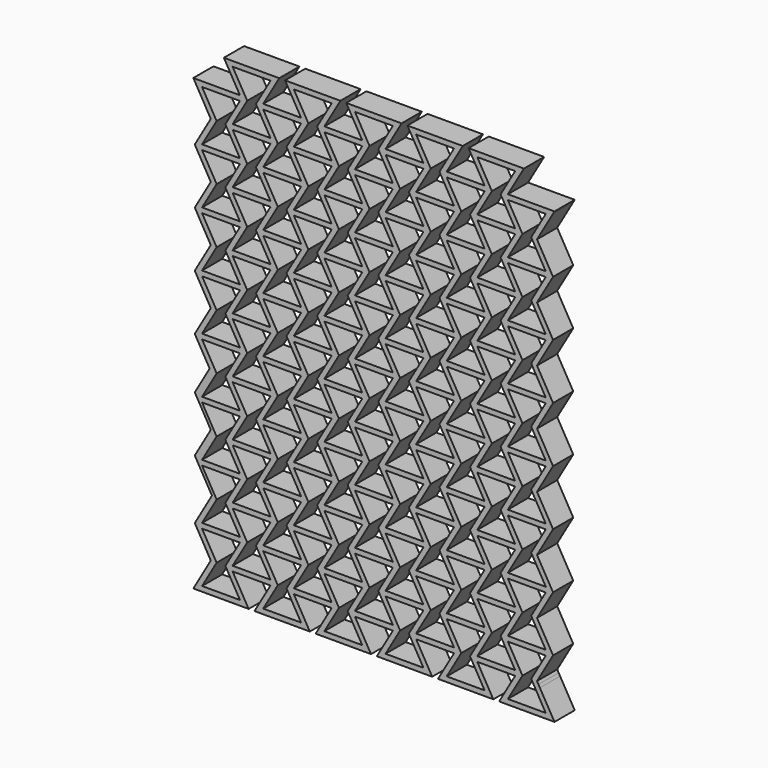
from build123d import *

# Parameters (mm, degrees)
F0_W     = 212.4550379813
F0_H     = 214.7212279961
F1_DEPTH = 10
F2_W     = 316.5591433644
F2_H     = 238.5154794902
F3_DEPTH = 50


# Not quite as in the source:
# - ends of sketch curves that miss each other by under 0.0002 mm in the source are joined


with BuildPart() as f1:
    # F0 (on Front) → F1 (new body)
    with BuildSketch(Plane.XZ):
        with Locations((69.8008518666, 93.7357270159)):
            Rectangle(F0_W, F0_H)
        Polygon((15, 0), (0, 0), (5.7735026919, 10), (0, 20), (15, 20), (9.2264973081, 10), align=None, mode=Mode.SUBTRACT)
        Polygon((15, 22), (0, 22), (5.7735026919, 32), (0, 42), (15, 42), (9.2264973081, 32), align=None, mode=Mode.SUBTRACT)
        Polygon((39.2264973081, 0), (24.2264973081, 0), (30, 10), (24.2264973081, 20), (39.2264973081, 20), (33.4529946162, 10), align=None, mode=Mode.SUBTRACT)
        Polygon((63.4529946162, 0), (48.4529946162, 0), (54.2264973081, 10), (48.4529946162, 20), (63.4529946162, 20), (57.6794919243, 10), align=None, mode=Mode.SUBTRACT)
        Polygon((27.1132486541, 11), (12.1132486541, 11), (17.8867513459, 21), (12.1132486541, 31), (27.1132486541, 31), (21.3397459622, 21), align=None, mode=Mode.SUBTRACT)
        Polygon((39.2264973081, 22), (24.2264973081, 22), (30, 32), (24.2264973081, 42), (39.2264973081, 42), (33.4529946162, 32), align=None, mode=Mode.SUBTRACT)
        Polygon((51.3397459622, 11), (36.3397459622, 11), (42.1132486541, 21), (36.3397459622, 31), (51.3397459622, 31), (45.5662432703, 21), align=None, mode=Mode.SUBTRACT)
        Polygon((75.5662432703, 11), (60.5662432703, 11), (66.3397459622, 21), (60.5662432703, 31), (75.5662432703, 31), (69.7927405784, 21), align=None, mode=Mode.SUBTRACT)
        Polygon((63.4529946162, 22), (48.4529946162, 22), (54.2264973081, 32), (48.4529946162, 42), (63.4529946162, 42), (57.6794919243, 32), align=None, mode=Mode.SUBTRACT)
        Polygon((15, 44), (0, 44), (5.7735026919, 54), (0, 64), (15, 64), (9.2264973081, 54), align=None, mode=Mode.SUBTRACT)
        Polygon((15, 66), (0, 66), (5.7735026919, 76), (0, 86), (15, 86), (9.2264973081, 76), align=None, mode=Mode.SUBTRACT)
        Polygon((27.1132486541, 33), (12.1132486541, 33), (17.8867513459, 43), (12.1132486541, 53), (27.1132486541, 53), (21.3397459622, 43), align=None, mode=Mode.SUBTRACT)
        Polygon((27.1132486541, 55), (12.1132486541, 55), (17.8867513459, 65), (12.1132486541, 75), (27.1132486541, 75), (21.3397459622, 65), align=None, mode=Mode.SUBTRACT)
        Polygon((39.2264973081, 44), (24.2264973081, 44), (30, 54), (24.2264973081, 64), (39.2264973081, 64), (33.4529946162, 54), align=None, mode=Mode.SUBTRACT)
        Polygon((51.3397459622, 33), (36.3397459622, 33), (42.1132486541, 43), (36.3397459622, 53), (51.3397459622, 53), (45.5662432703, 43), align=None, mode=Mode.SUBTRACT)
        Polygon((75.5662432703, 33), (60.5662432703, 33), (66.3397459622, 43), (60.5662432703, 53), (75.5662432703, 53), (69.7927405784, 43), align=None, mode=Mode.SUBTRACT)
        Polygon((63.4529946162, 44), (48.4529946162, 44), (54.2264973081, 54), (48.4529946162, 64), (63.4529946162, 64), (57.6794919243, 54), align=None, mode=Mode.SUBTRACT)
        Polygon((51.3397459622, 55), (36.3397459622, 55), (42.1132486541, 65), (36.3397459622, 75), (51.3397459622, 75), (45.5662432703, 65), align=None, mode=Mode.SUBTRACT)
        Polygon((75.5662432703, 55), (60.5662432703, 55), (66.3397459622, 65), (60.5662432703, 75), (75.5662432703, 75), (69.7927405784, 65), align=None, mode=Mode.SUBTRACT)
        Polygon((39.2264973081, 66), (24.2264973081, 66), (30, 76), (24.2264973081, 86), (39.2264973081, 86), (33.4529946162, 76), align=None, mode=Mode.SUBTRACT)
        Polygon((27.1132486541, 77), (12.1132486541, 77), (17.8867513459, 87), (12.1132486541, 97), (27.1132486541, 97), (21.3397459622, 87), align=None, mode=Mode.SUBTRACT)
        Polygon((63.4529946162, 66), (48.4529946162, 66), (54.2264973081, 76), (48.4529946162, 86), (63.4529946162, 86), (57.6794919243, 76), align=None, mode=Mode.SUBTRACT)
        Polygon((51.3397459622, 77), (36.3397459622, 77), (42.1132486541, 87), (36.3397459622, 97), (51.3397459622, 97), (45.5662432703, 87), align=None, mode=Mode.SUBTRACT)
        Polygon((75.5662432703, 77), (60.5662432703, 77), (66.3397459622, 87), (60.5662432703, 97), (75.5662432703, 97), (69.7927405784, 87), align=None, mode=Mode.SUBTRACT)
        Polygon((87.6794919243, 0), (72.6794919243, 0), (78.4529946162, 10), (72.6794919243, 20), (87.6794919243, 20), (81.9059892324, 10), align=None, mode=Mode.SUBTRACT)
        Polygon((111.9059892324, 0), (96.9059892324, 0), (102.6794919243, 10), (96.9059892324, 20), (111.9059892324, 20), (106.1324865405, 10), align=None, mode=Mode.SUBTRACT)
        Polygon((99.7927405784, 11), (84.7927405784, 11), (90.5662432703, 21), (84.7927405784, 31), (99.7927405784, 31), (94.0192378865, 21), align=None, mode=Mode.SUBTRACT)
        Polygon((87.6794919243, 22), (72.6794919243, 22), (78.4529946162, 32), (72.6794919243, 42), (87.6794919243, 42), (81.9059892324, 32), align=None, mode=Mode.SUBTRACT)
        Polygon((124.0192378865, 11), (109.0192378865, 11), (114.7927405784, 21), (109.0192378865, 31), (124.0192378865, 31), (118.2457351946, 21), align=None, mode=Mode.SUBTRACT)
        Polygon((111.9059892324, 22), (96.9059892324, 22), (102.6794919243, 32), (96.9059892324, 42), (111.9059892324, 42), (106.1324865405, 32), align=None, mode=Mode.SUBTRACT)
        Polygon((136.1324865405, 0), (121.1324865405, 0), (126.9059892324, 10), (121.1324865405, 20), (136.1324865405, 20), (130.3589838486, 10), align=None, mode=Mode.SUBTRACT)
        Polygon((148.2457351946, 11), (133.2457351946, 11), (139.0192378865, 21), (133.2457351946, 31), (148.2457351946, 31), (142.4722325027, 21), align=None, mode=Mode.SUBTRACT)
        Polygon((136.1324865405, 22), (121.1324865405, 22), (126.9059892324, 32), (121.1324865405, 42), (136.1324865405, 42), (130.3589838486, 32), align=None, mode=Mode.SUBTRACT)
        Polygon((99.7927405784, 33), (84.7927405784, 33), (90.5662432703, 43), (84.7927405784, 53), (99.7927405784, 53), (94.0192378865, 43), align=None, mode=Mode.SUBTRACT)
        Polygon((87.6794919243, 44), (72.6794919243, 44), (78.4529946162, 54), (72.6794919243, 64), (87.6794919243, 64), (81.9059892324, 54), align=None, mode=Mode.SUBTRACT)
        Polygon((99.7927405784, 55), (84.7927405784, 55), (90.5662432703, 65), (84.7927405784, 75), (99.7927405784, 75), (94.0192378865, 65), align=None, mode=Mode.SUBTRACT)
        Polygon((124.0192378865, 33), (109.0192378865, 33), (114.7927405784, 43), (109.0192378865, 53), (124.0192378865, 53), (118.2457351946, 43), align=None, mode=Mode.SUBTRACT)
        Polygon((111.9059892324, 44), (96.9059892324, 44), (102.6794919243, 54), (96.9059892324, 64), (111.9059892324, 64), (106.1324865405, 54), align=None, mode=Mode.SUBTRACT)
        Polygon((124.0192378865, 55), (109.0192378865, 55), (114.7927405784, 65), (109.0192378865, 75), (124.0192378865, 75), (118.2457351946, 65), align=None, mode=Mode.SUBTRACT)
        Polygon((87.6794919243, 66), (72.6794919243, 66), (78.4529946162, 76), (72.6794919243, 86), (87.6794919243, 86), (81.9059892324, 76), align=None, mode=Mode.SUBTRACT)
        Polygon((99.7927405784, 77), (84.7927405784, 77), (90.5662432703, 87), (84.7927405784, 97), (99.7927405784, 97), (94.0192378865, 87), align=None, mode=Mode.SUBTRACT)
        Polygon((111.9059892324, 66), (96.9059892324, 66), (102.6794919243, 76), (96.9059892324, 86), (111.9059892324, 86), (106.1324865405, 76), align=None, mode=Mode.SUBTRACT)
        Polygon((124.0192378865, 77), (109.0192378865, 77), (114.7927405784, 87), (109.0192378865, 97), (124.0192378865, 97), (118.2457351946, 87), align=None, mode=Mode.SUBTRACT)
        Polygon((148.2457351946, 33), (133.2457351946, 33), (139.0192378865, 43), (133.2457351946, 53), (148.2457351946, 53), (142.4722325027, 43), align=None, mode=Mode.SUBTRACT)
        Polygon((136.1324865405, 44), (121.1324865405, 44), (126.9059892324, 54), (121.1324865405, 64), (136.1324865405, 64), (130.3589838486, 54), align=None, mode=Mode.SUBTRACT)
        Polygon((148.2457351946, 55), (133.2457351946, 55), (139.0192378865, 65), (133.2457351946, 75), (148.2457351946, 75), (142.4722325027, 65), align=None, mode=Mode.SUBTRACT)
        Polygon((136.1324865405, 66), (121.1324865405, 66), (126.9059892324, 76), (121.1324865405, 86), (136.1324865405, 86), (130.3589838486, 76), align=None, mode=Mode.SUBTRACT)
        Polygon((148.2457351946, 77), (133.2457351946, 77), (139.0192378865, 87), (133.2457351946, 97), (148.2457351946, 97), (142.4722325027, 87), align=None, mode=Mode.SUBTRACT)
        Polygon((15, 88), (0, 88), (5.7735026919, 98), (0, 108), (15, 108), (9.2264973081, 98), align=None, mode=Mode.SUBTRACT)
        Polygon((15, 110), (0, 110), (5.7735026919, 120), (0, 130), (15, 130), (9.2264973081, 120), align=None, mode=Mode.SUBTRACT)
        Polygon((15, 132), (0, 132), (5.7735026919, 142), (0, 152), (15, 152), (9.2264973081, 142), align=None, mode=Mode.SUBTRACT)
        Polygon((39.2264973081, 88), (24.2264973081, 88), (30, 98), (24.2264973081, 108), (39.2264973081, 108), (33.4529946162, 98), align=None, mode=Mode.SUBTRACT)
        Polygon((27.1132486541, 99), (12.1132486541, 99), (17.8867513459, 109), (12.1132486541, 119), (27.1132486541, 119), (21.3397459622, 109), align=None, mode=Mode.SUBTRACT)
        Polygon((39.2264973081, 110), (24.2264973081, 110), (30, 120), (24.2264973081, 130), (39.2264973081, 130), (33.4529946162, 120), align=None, mode=Mode.SUBTRACT)
        Polygon((63.4529946162, 88), (48.4529946162, 88), (54.2264973081, 98), (48.4529946162, 108), (63.4529946162, 108), (57.6794919243, 98), align=None, mode=Mode.SUBTRACT)
        Polygon((51.3397459622, 99), (36.3397459622, 99), (42.1132486541, 109), (36.3397459622, 119), (51.3397459622, 119), (45.5662432703, 109), align=None, mode=Mode.SUBTRACT)
        Polygon((63.4529946162, 110), (48.4529946162, 110), (54.2264973081, 120), (48.4529946162, 130), (63.4529946162, 130), (57.6794919243, 120), align=None, mode=Mode.SUBTRACT)
        Polygon((75.5662432703, 99), (60.5662432703, 99), (66.3397459622, 109), (60.5662432703, 119), (75.5662432703, 119), (69.7927405784, 109), align=None, mode=Mode.SUBTRACT)
        Polygon((27.1132486541, 121), (12.1132486541, 121), (17.8867513459, 131), (12.1132486541, 141), (27.1132486541, 141), (21.3397459622, 131), align=None, mode=Mode.SUBTRACT)
        Polygon((39.2264973081, 132), (24.2264973081, 132), (30, 142), (24.2264973081, 152), (39.2264973081, 152), (33.4529946162, 142), align=None, mode=Mode.SUBTRACT)
        Polygon((51.3397459622, 121), (36.3397459622, 121), (42.1132486541, 131), (36.3397459622, 141), (51.3397459622, 141), (45.5662432703, 131), align=None, mode=Mode.SUBTRACT)
        Polygon((75.5662432703, 121), (60.5662432703, 121), (66.3397459622, 131), (60.5662432703, 141), (75.5662432703, 141), (69.7927405784, 131), align=None, mode=Mode.SUBTRACT)
        Polygon((63.4529946162, 132), (48.4529946162, 132), (54.2264973081, 142), (48.4529946162, 152), (63.4529946162, 152), (57.6794919243, 142), align=None, mode=Mode.SUBTRACT)
        Polygon((15, 154), (0, 154), (5.7735026919, 164), (0, 174), (15, 174), (9.2264973081, 164), align=None, mode=Mode.SUBTRACT)
        Polygon((27.1132486541, 143), (12.1132486541, 143), (17.8867513459, 153), (12.1132486541, 163), (27.1132486541, 163), (21.3397459622, 153), align=None, mode=Mode.SUBTRACT)
        Polygon((39.2264973081, 154), (24.2264973081, 154), (30, 164), (24.2264973081, 174), (39.2264973081, 174), (33.4529946162, 164), align=None, mode=Mode.SUBTRACT)
        Polygon((51.3397459622, 143), (36.3397459622, 143), (42.1132486541, 153), (36.3397459622, 163), (51.3397459622, 163), (45.5662432703, 153), align=None, mode=Mode.SUBTRACT)
        Polygon((75.5662432703, 143), (60.5662432703, 143), (66.3397459622, 153), (60.5662432703, 163), (75.5662432703, 163), (69.7927405784, 153), align=None, mode=Mode.SUBTRACT)
        Polygon((63.4529946162, 154), (48.4529946162, 154), (54.2264973081, 164), (48.4529946162, 174), (63.4529946162, 174), (57.6794919243, 164), align=None, mode=Mode.SUBTRACT)
        Polygon((27.1132486541, 165), (12.1132486541, 165), (17.8867513459, 175), (12.1132486541, 185), (27.1132486541, 185), (21.3397459622, 175), align=None, mode=Mode.SUBTRACT)
        Polygon((51.3397459622, 165), (36.3397459622, 165), (42.1132486541, 175), (36.3397459622, 185), (51.3397459622, 185), (45.5662432703, 175), align=None, mode=Mode.SUBTRACT)
        Polygon((75.5662432703, 165), (60.5662432703, 165), (66.3397459622, 175), (60.5662432703, 185), (75.5662432703, 185), (69.7927405784, 175), align=None, mode=Mode.SUBTRACT)
        Polygon((87.6794919243, 88), (72.6794919243, 88), (78.4529946162, 98), (72.6794919243, 108), (87.6794919243, 108), (81.9059892324, 98), align=None, mode=Mode.SUBTRACT)
        Polygon((87.6794919243, 110), (72.6794919243, 110), (78.4529946162, 120), (72.6794919243, 130), (87.6794919243, 130), (81.9059892324, 120), align=None, mode=Mode.SUBTRACT)
        Polygon((99.7927405784, 99), (84.7927405784, 99), (90.5662432703, 109), (84.7927405784, 119), (99.7927405784, 119), (94.0192378865, 109), align=None, mode=Mode.SUBTRACT)
        Polygon((111.9059892324, 88), (96.9059892324, 88), (102.6794919243, 98), (96.9059892324, 108), (111.9059892324, 108), (106.1324865405, 98), align=None, mode=Mode.SUBTRACT)
        Polygon((111.9059892324, 110), (96.9059892324, 110), (102.6794919243, 120), (96.9059892324, 130), (111.9059892324, 130), (106.1324865405, 120), align=None, mode=Mode.SUBTRACT)
        Polygon((124.0192378865, 99), (109.0192378865, 99), (114.7927405784, 109), (109.0192378865, 119), (124.0192378865, 119), (118.2457351946, 109), align=None, mode=Mode.SUBTRACT)
        Polygon((99.7927405784, 121), (84.7927405784, 121), (90.5662432703, 131), (84.7927405784, 141), (99.7927405784, 141), (94.0192378865, 131), align=None, mode=Mode.SUBTRACT)
        Polygon((87.6794919243, 132), (72.6794919243, 132), (78.4529946162, 142), (72.6794919243, 152), (87.6794919243, 152), (81.9059892324, 142), align=None, mode=Mode.SUBTRACT)
        Polygon((124.0192378865, 121), (109.0192378865, 121), (114.7927405784, 131), (109.0192378865, 141), (124.0192378865, 141), (118.2457351946, 131), align=None, mode=Mode.SUBTRACT)
        Polygon((111.9059892324, 132), (96.9059892324, 132), (102.6794919243, 142), (96.9059892324, 152), (111.9059892324, 152), (106.1324865405, 142), align=None, mode=Mode.SUBTRACT)
        Polygon((136.1324865405, 88), (121.1324865405, 88), (126.9059892324, 98), (121.1324865405, 108), (136.1324865405, 108), (130.3589838486, 98), align=None, mode=Mode.SUBTRACT)
        Polygon((136.1324865405, 110), (121.1324865405, 110), (126.9059892324, 120), (121.1324865405, 130), (136.1324865405, 130), (130.3589838486, 120), align=None, mode=Mode.SUBTRACT)
        Polygon((148.2457351946, 99), (133.2457351946, 99), (139.0192378865, 109), (133.2457351946, 119), (148.2457351946, 119), (142.4722325027, 109), align=None, mode=Mode.SUBTRACT)
        Polygon((148.2457351946, 121), (133.2457351946, 121), (139.0192378865, 131), (133.2457351946, 141), (148.2457351946, 141), (142.4722325027, 131), align=None, mode=Mode.SUBTRACT)
        Polygon((136.1324865405, 132), (121.1324865405, 132), (126.9059892324, 142), (121.1324865405, 152), (136.1324865405, 152), (130.3589838486, 142), align=None, mode=Mode.SUBTRACT)
        Polygon((99.7927405784, 143), (84.7927405784, 143), (90.5662432703, 153), (84.7927405784, 163), (99.7927405784, 163), (94.0192378865, 153), align=None, mode=Mode.SUBTRACT)
        Polygon((87.6794919243, 154), (72.6794919243, 154), (78.4529946162, 164), (72.6794919243, 174), (87.6794919243, 174), (81.9059892324, 164), align=None, mode=Mode.SUBTRACT)
        Polygon((124.0192378865, 143), (109.0192378865, 143), (114.7927405784, 153), (109.0192378865, 163), (124.0192378865, 163), (118.2457351946, 153), align=None, mode=Mode.SUBTRACT)
        Polygon((111.9059892324, 154), (96.9059892324, 154), (102.6794919243, 164), (96.9059892324, 174), (111.9059892324, 174), (106.1324865405, 164), align=None, mode=Mode.SUBTRACT)
        Polygon((99.7927405784, 165), (84.7927405784, 165), (90.5662432703, 175), (84.7927405784, 185), (99.7927405784, 185), (94.0192378865, 175), align=None, mode=Mode.SUBTRACT)
        Polygon((124.0192378865, 165), (109.0192378865, 165), (114.7927405784, 175), (109.0192378865, 185), (124.0192378865, 185), (118.2457351946, 175), align=None, mode=Mode.SUBTRACT)
        Polygon((148.2457351946, 143), (133.2457351946, 143), (139.0192378865, 153), (133.2457351946, 163), (148.2457351946, 163), (142.4722325027, 153), align=None, mode=Mode.SUBTRACT)
        Polygon((136.1324865405, 154), (121.1324865405, 154), (126.9059892324, 164), (121.1324865405, 174), (136.1324865405, 174), (130.3589838486, 164), align=None, mode=Mode.SUBTRACT)
    extrude(amount=F1_DEPTH)

    # F2 (on face) → F3 (cut)
    with BuildSketch(Plane.XZ.offset(10)):
        with Locations((79.4346891344, 93.9047122374)):
            Rectangle(F2_W, F2_H)
        Polygon((27.1132486541, 9), (12.1132486541, 9), (18.4641016151, -2), (-3.4641016151, -2), (2.8867513459, 9), (3.4641016151, 10), (0.8151336812, 14.5881470491), (-2.8867513459, 21), (3.9156507662, 32.7821060717), (-2.8867513459, 44.5642121434), (3.4641016151, 55.5642121434), (-2.8867513459, 66.5642121434), (3.0125524641, 76.7821060717), (-2.8867513459, 87), (3.4641016151, 98), (-2.8867513459, 109), (3.4641016151, 120), (-2.8867513459, 131), (3.4641016151, 142), (-2.8867513459, 153), (3.4641016151, 164), (-0.2377831429, 170.4118524846), (-2.8867513459, 175), (-3.4641005384, 176), (15, 176), (8.6491470389, 187), (30.5773502692, 187), (24.2264973081, 176), (39.2264973081, 176), (32.875644347, 187), (54.8038475773, 187), (48.4529946162, 176), (63.4529946162, 176), (57.1021416551, 187), (79.0303448854, 187), (72.6794919243, 176), (87.6794919243, 176), (81.3286389632, 187), (103.2568421935, 187), (96.9059892324, 176), (111.9059892324, 176), (105.5551362713, 187), (127.4833395016, 187), (121.1324865405, 176), (136.1324865405, 176), (139.5965881557, 176), (139.0192378865, 175), (132.6683849254, 164), (139.0192378865, 153), (132.6683849254, 142), (139.0192378865, 131), (132.6683849254, 120), (139.0192378865, 109), (132.6683849254, 98), (139.0192378865, 87), (132.6683849254, 76), (139.0192378865, 65), (132.6683849254, 54), (139.0192378865, 43), (132.6683849254, 32), (139.0192378865, 21), (132.6683849254, 10), (133.2457351946, 9), (133.8058562328, 8.0298419035), (139.5965881557, -2), (117.6683849254, -2), (124.0192378865, 9), (109.0192378865, 9), (115.3700908476, -2), (93.4418876173, -2), (99.7927405784, 9), (84.7927405784, 9), (91.1435935394, -2), (69.2153903092, -2), (75.5662432703, 9), (60.5662432703, 9), (66.9170962313, -2), (44.9888930011, -2), (51.3397459622, 9), (36.3397459622, 9), (42.6905989232, -2), (20.762395693, -2), align=None, mode=Mode.SUBTRACT)
    extrude(amount=-F3_DEPTH, mode=Mode.SUBTRACT)


solid = f1.part
